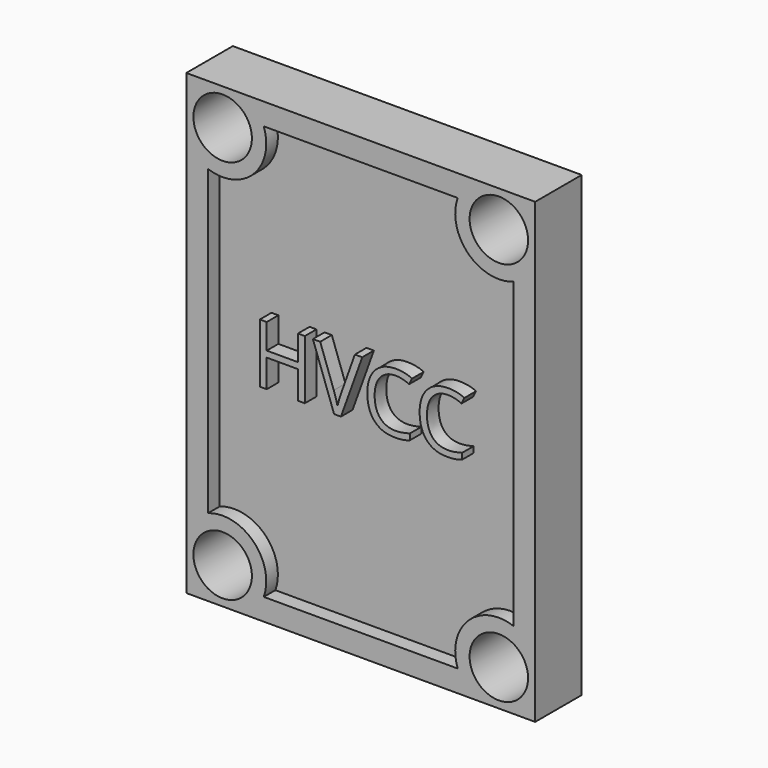
from build123d import *

# Parameters (mm, degrees)
F0_W         = 48
F0_H         = 63
F0_R         = 4.025
F0_TEXT_SIZE = 11.4075218347
F1_DEPTH     = 8
F3_DEPTH     = 2
F4_DEPTH     = 8


# Not quite as in the source:
# - Text() gives the source's letters only with a copy of the font that has no kerning and outlines rounded to 1/6400 em; it was checked with that copy


with BuildPart() as f1:
    # F0 (on Front) → F1 (new body)
    with BuildSketch(Plane.XZ):
        with Locations((-24, -31.5)):
            Rectangle(F0_W, F0_H)
        with Locations((-43, -58)):
            Circle(F0_R, mode=Mode.SUBTRACT)
        with Locations((-5, -58)):
            Circle(F0_R, mode=Mode.SUBTRACT)
        with Locations((-43, -5)):
            Circle(F0_R, mode=Mode.SUBTRACT)
        with BuildLine():
            Line((-45, -50), (-45, -13))
            ThreePointArc((-45, -13), (-44.4142135624, -11.5857864376), (-43, -11))
            ThreePointArc((-43, -11), (-38.7573593129, -9.2426406871), (-37, -5))
            ThreePointArc((-37, -5), (-36.4142135624, -3.5857864376), (-35, -3))
            Line((-35, -3), (-13, -3))
            ThreePointArc((-13, -3), (-11.5857864376, -3.5857864376), (-11, -5))
            ThreePointArc((-11, -5), (-9.2426406871, -9.2426406871), (-5, -11))
            ThreePointArc((-5, -11), (-3.5857864376, -11.5857864376), (-3, -13))
            Line((-3, -13), (-3, -50))
            ThreePointArc((-3, -50), (-3.5857864376, -51.4142135624), (-5, -52))
            ThreePointArc((-5, -52), (-9.2426406871, -53.7573593129), (-11, -58))
            ThreePointArc((-11, -58), (-11.5857864376, -59.4142135624), (-13, -60))
            Line((-13, -60), (-35, -60))
            ThreePointArc((-35, -60), (-36.4142135624, -59.4142135624), (-37, -58))
            ThreePointArc((-37, -58), (-38.7573593129, -53.7573593129), (-43, -52))
            ThreePointArc((-43, -52), (-44.4142135624, -51.4142135624), (-45, -50))
        make_face(mode=Mode.SUBTRACT)
        with Locations((-5, -5)):
            Circle(F0_R, mode=Mode.SUBTRACT)
        with BuildLine():
            ThreePointArc((-43, -11), (-44.4142135624, -11.5857864376), (-45, -13))
            Line((-45, -13), (-45, -50))
            ThreePointArc((-45, -50), (-44.4142135624, -51.4142135624), (-43, -52))
            ThreePointArc((-43, -52), (-38.7573593129, -53.7573593129), (-37, -58))
            ThreePointArc((-37, -58), (-36.4142135624, -59.4142135624), (-35, -60))
            Line((-35, -60), (-13, -60))
            ThreePointArc((-13, -60), (-11.5857864376, -59.4142135624), (-11, -58))
            ThreePointArc((-11, -58), (-9.2426406871, -53.7573593129), (-5, -52))
            ThreePointArc((-5, -52), (-3.5857864376, -51.4142135624), (-3, -50))
            Line((-3, -50), (-3, -13))
            ThreePointArc((-3, -13), (-3.5857864376, -11.5857864376), (-5, -11))
            ThreePointArc((-5, -11), (-9.2426406871, -9.2426406871), (-11, -5))
            ThreePointArc((-11, -5), (-11.5857864376, -3.5857864376), (-13, -3))
            Line((-13, -3), (-35, -3))
            ThreePointArc((-35, -3), (-36.4142135624, -3.5857864376), (-37, -5))
            ThreePointArc((-37, -5), (-38.7573593129, -9.2426406871), (-43, -11))
        make_face()
        Polygon((-31.6974036005, -26.5695145862), (-31.6974036005, -34.713415721), (-32.6438714277, -34.713415721), (-32.6438714277, -30.8812013546), (-36.9341690927, -30.8812013546), (-36.9341690927, -34.713415721), (-37.88063692, -34.713415721), (-37.88063692, -26.5695145862), (-36.9341690927, -26.5695145862), (-36.9341690927, -30.0345493435), (-32.6438714277, -30.0345493435), (-32.6438714277, -26.5695145862), align=None, mode=Mode.SUBTRACT)
        with BuildLine():
            Line((-26.6727467174, -31.8062800784), (-24.8118947181, -26.5695145862))
            Line((-24.8118947181, -26.5695145862), (-23.7941298794, -26.5695145862))
            Line((-23.7941298794, -26.5695145862), (-26.7280019013, -34.713415721))
            Line((-26.7280019013, -34.713415721), (-27.6637751768, -34.713415721))
            Line((-27.6637751768, -34.713415721), (-30.5833877963, -26.5695145862))
            Line((-30.5833877963, -26.5695145862), (-29.5798823599, -26.5695145862))
            Line((-29.5798823599, -26.5695145862), (-27.7083358089, -31.8383637336))
            add(Edge.make_bspline(
                [(-27.7083358089, -31.8383637336), (-27.385716832, -32.7474006298), (-27.1967797516, -33.6047471927)],
                knots=[0, 0, 0, 1, 1, 1], degree=2))
            add(Edge.make_bspline(
                [(-27.1967797516, -33.6047471927), (-26.9953656943, -32.7028399976), (-26.6727467174, -31.8062800784)],
                knots=[0, 0, 0, 1, 1, 1], degree=2))
        make_face(mode=Mode.SUBTRACT)
        with BuildLine():
            add(Edge.make_bspline(
                [(-17.3381854911, -27.7334382984), (-18.2632642148, -27.3003089537), (-19.1883429386, -27.3003089537)],
                knots=[0, 0, 0, 1, 1, 1], degree=2))
            add(Edge.make_bspline(
                [(-19.1883429386, -27.3003089537), (-20.5305091795, -27.3003089537), (-21.3076466045, -28.194195235)],
                knots=[0, 0, 0, 1, 1, 1], degree=2))
            add(Edge.make_bspline(
                [(-21.3076466045, -28.194195235), (-22.0847840295, -29.0880815162), (-22.0847840295, -30.6423563662)],
                knots=[0, 0, 0, 1, 1, 1], degree=2))
            add(Edge.make_bspline(
                [(-22.0847840295, -30.6423563662), (-22.0847840295, -32.2394094231), (-21.3352741964, -33.1119066009)],
                knots=[0, 0, 0, 1, 1, 1], degree=2))
            add(Edge.make_bspline(
                [(-21.3352741964, -33.1119066009), (-20.5857643634, -33.9844037787), (-19.1990374903, -33.9844037787)],
                knots=[0, 0, 0, 1, 1, 1], degree=2))
            add(Edge.make_bspline(
                [(-19.1990374903, -33.9844037787), (-18.3470382033, -33.9844037787), (-17.2544115026, -33.6778266294)],
                knots=[0, 0, 0, 1, 1, 1], degree=2))
            Line((-17.2544115026, -33.6778266294), (-17.2544115026, -34.5066543877))
            add(Edge.make_bspline(
                [(-17.2544115026, -34.5066543877), (-18.1010635138, -34.8257085141), (-19.3434139386, -34.8257085141)],
                knots=[0, 0, 0, 1, 1, 1], degree=2))
            add(Edge.make_bspline(
                [(-19.3434139386, -34.8257085141), (-21.1418810528, -34.8257085141), (-22.1195413226, -33.7330818133)],
                knots=[0, 0, 0, 1, 1, 1], degree=2))
            add(Edge.make_bspline(
                [(-22.1195413226, -33.7330818133), (-23.0972015923, -32.6404551126), (-23.0972015923, -30.6298793892)],
                knots=[0, 0, 0, 1, 1, 1], degree=2))
            add(Edge.make_bspline(
                [(-23.0972015923, -30.6298793892), (-23.0972015923, -29.3714871368), (-22.6266413166, -28.4250193096)],
                knots=[0, 0, 0, 1, 1, 1], degree=2))
            add(Edge.make_bspline(
                [(-22.6266413166, -28.4250193096), (-22.1560810409, -27.4785514824), (-21.2675420355, -26.9661042125)],
                knots=[0, 0, 0, 1, 1, 1], degree=2))
            add(Edge.make_bspline(
                [(-21.2675420355, -26.9661042125), (-20.3790030301, -26.4536569425), (-19.1758659616, -26.4536569425)],
                knots=[0, 0, 0, 1, 1, 1], degree=2))
            add(Edge.make_bspline(
                [(-19.1758659616, -26.4536569425), (-17.8960846058, -26.4536569425), (-16.9371398016, -26.9206523677)],
                knots=[0, 0, 0, 1, 1, 1], degree=2))
            Line((-16.9371398016, -26.9206523677), (-17.3381854911, -27.7334382984))
        make_face(mode=Mode.SUBTRACT)
        with BuildLine():
            add(Edge.make_bspline(
                [(-10.1407521835, -27.7334382984), (-11.0658309073, -27.3003089537), (-11.990909631, -27.3003089537)],
                knots=[0, 0, 0, 1, 1, 1], degree=2))
            add(Edge.make_bspline(
                [(-11.990909631, -27.3003089537), (-13.3330758719, -27.3003089537), (-14.1102132969, -28.194195235)],
                knots=[0, 0, 0, 1, 1, 1], degree=2))
            add(Edge.make_bspline(
                [(-14.1102132969, -28.194195235), (-14.8873507219, -29.0880815162), (-14.8873507219, -30.6423563662)],
                knots=[0, 0, 0, 1, 1, 1], degree=2))
            add(Edge.make_bspline(
                [(-14.8873507219, -30.6423563662), (-14.8873507219, -32.2394094231), (-14.1378408888, -33.1119066009)],
                knots=[0, 0, 0, 1, 1, 1], degree=2))
            add(Edge.make_bspline(
                [(-14.1378408888, -33.1119066009), (-13.3883310558, -33.9844037787), (-12.0016041828, -33.9844037787)],
                knots=[0, 0, 0, 1, 1, 1], degree=2))
            add(Edge.make_bspline(
                [(-12.0016041828, -33.9844037787), (-11.1496048957, -33.9844037787), (-10.056978195, -33.6778266294)],
                knots=[0, 0, 0, 1, 1, 1], degree=2))
            Line((-10.056978195, -33.6778266294), (-10.056978195, -34.5066543877))
            add(Edge.make_bspline(
                [(-10.056978195, -34.5066543877), (-10.9036302062, -34.8257085141), (-12.145980631, -34.8257085141)],
                knots=[0, 0, 0, 1, 1, 1], degree=2))
            add(Edge.make_bspline(
                [(-12.145980631, -34.8257085141), (-13.9444477452, -34.8257085141), (-14.922108015, -33.7330818133)],
                knots=[0, 0, 0, 1, 1, 1], degree=2))
            add(Edge.make_bspline(
                [(-14.922108015, -33.7330818133), (-15.8997682847, -32.6404551126), (-15.8997682847, -30.6298793892)],
                knots=[0, 0, 0, 1, 1, 1], degree=2))
            add(Edge.make_bspline(
                [(-15.8997682847, -30.6298793892), (-15.8997682847, -29.3714871368), (-15.429208009, -28.4250193096)],
                knots=[0, 0, 0, 1, 1, 1], degree=2))
            add(Edge.make_bspline(
                [(-15.429208009, -28.4250193096), (-14.9586477333, -27.4785514824), (-14.0701087279, -26.9661042125)],
                knots=[0, 0, 0, 1, 1, 1], degree=2))
            add(Edge.make_bspline(
                [(-14.0701087279, -26.9661042125), (-13.1815697225, -26.4536569425), (-11.978432654, -26.4536569425)],
                knots=[0, 0, 0, 1, 1, 1], degree=2))
            add(Edge.make_bspline(
                [(-11.978432654, -26.4536569425), (-10.6986512982, -26.4536569425), (-9.739706494, -26.9206523677)],
                knots=[0, 0, 0, 1, 1, 1], degree=2))
            Line((-9.739706494, -26.9206523677), (-10.1407521835, -27.7334382984))
        make_face(mode=Mode.SUBTRACT)
        with Locations((-39, -34.713415721)):
            Text('HVCC', F0_TEXT_SIZE, font='Open Sans', text_align=(TextAlign.LEFT, TextAlign.BOTTOM))
    extrude(amount=F1_DEPTH)

    # F2 (on face) → F3 (cut)
    with BuildSketch(Plane.XZ.offset(8)):
        with BuildLine():
            ThreePointArc((-37.3431457505, -3), (-38.7573593129, -9.2426406871), (-45, -10.6568542495))
            Line((-45, -10.6568542495), (-45, -52.3431457505))
            ThreePointArc((-45, -52.3431457505), (-38.7573593129, -53.7573593129), (-37.3431457505, -60))
            Line((-37.3431457505, -60), (-10.6568542495, -60))
            ThreePointArc((-10.6568542495, -60), (-9.2426406871, -53.7573593129), (-3, -52.3431457505))
            Line((-3, -52.3431457505), (-3, -10.6568542495))
            ThreePointArc((-3, -10.6568542495), (-9.2426406871, -9.2426406871), (-10.6568542495, -3))
            Line((-10.6568542495, -3), (-37.3431457505, -3))
        make_face()
    extrude(amount=-F3_DEPTH, mode=Mode.SUBTRACT)

    # F0 (on Front) → F4 (join)
    with BuildSketch(Plane.XZ):
        with Locations((-39, -34.713415721)):
            Text('HVCC', F0_TEXT_SIZE, font='Open Sans', text_align=(TextAlign.LEFT, TextAlign.BOTTOM))
    extrude(amount=F4_DEPTH)


solid = f1.part
